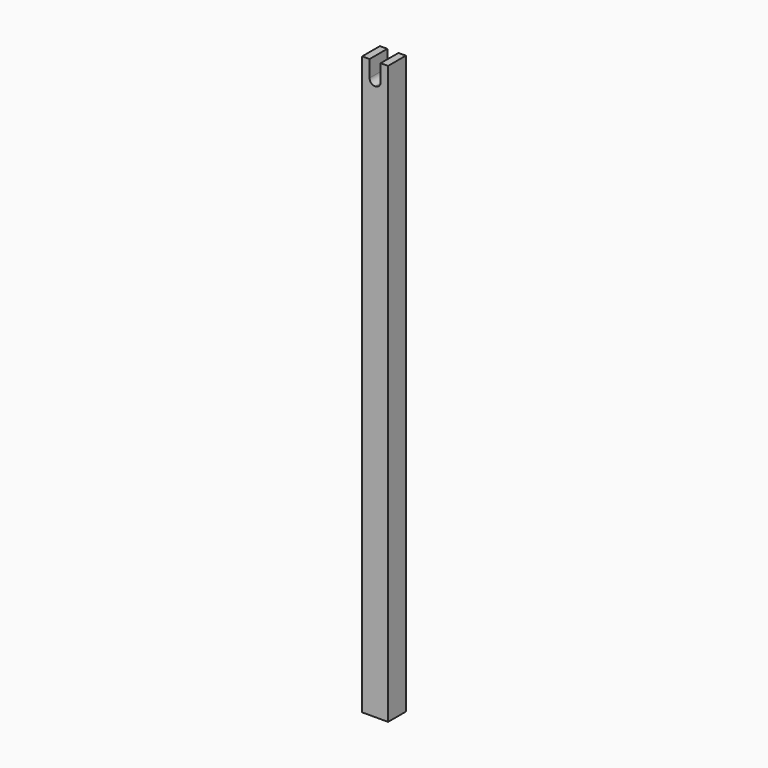
from build123d import *

# Parameters (mm, degrees)
F0_W     = 44.45
F0_H     = 990.6
F1_DEPTH = 38.1
F2_W     = 19.05
F2_H     = 38.1
F3_DEPTH = 38.101
F4_R     = 9.52499


# Not quite as in the source:
# - a fillet or chamfer is up to 0.001 mm smaller than in the source, because OpenCascade refuses the exact size


with BuildPart() as f1:
    # F0 (on Front) → F1 (new body)
    with BuildSketch(Plane.XZ):
        with Locations((22.225, 495.3)):
            Rectangle(F0_W, F0_H)
    extrude(amount=F1_DEPTH)

    # F2 (on face) → F3 (cut, through all)
    with BuildSketch(Plane.XZ.offset(38.1)):
        with Locations((22.225, 971.55)):
            Rectangle(F2_W, F2_H)
    extrude(amount=-F3_DEPTH, mode=Mode.SUBTRACT)

    # F4 (radius 9.525 in the source; OpenCascade refuses exactly that, so slightly less here)
    f4_edges = [f1.edges().sort_by_distance(p)[0] for p in [
        (12.7, -19.05, 952.5),
        (31.75, -19.05, 952.5),
    ]]
    fillet(f4_edges, radius=F4_R)


solid = f1.part
